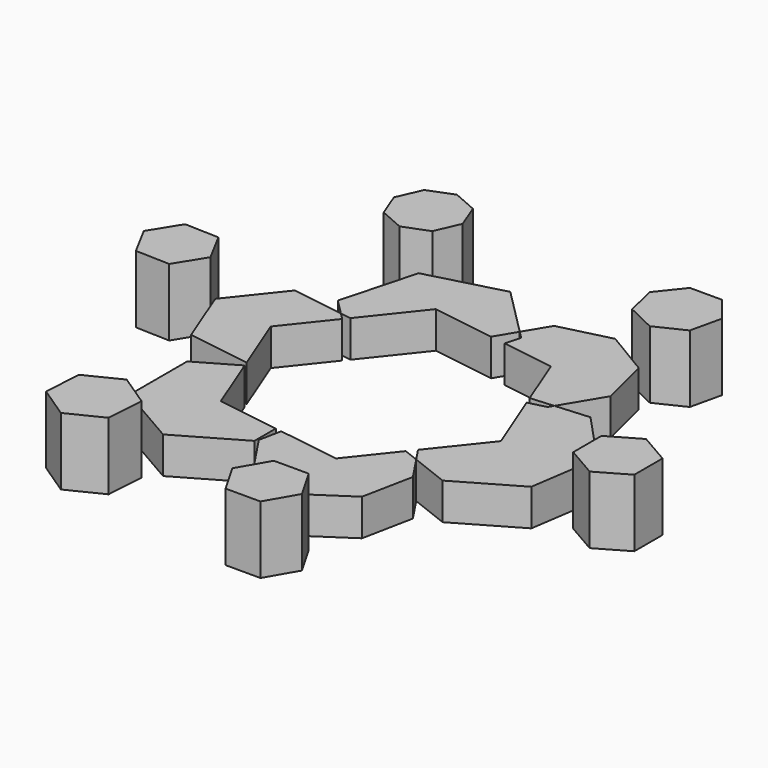
from build123d import *

# Parameters (mm, degrees)
F1_DEPTH = 25
F5_DEPTH = 46


# Not quite as in the source:
# - the program builds the solid bodies; features that only make, move or delete a surface that nothing else refers to are left out


with BuildPart() as f1:
    # F0 (on Top) → F1 (new body)
    with BuildSketch(Plane.XY):
        Polygon((222.1852089025, -548.7398207486), (222.1852089025, -530.5067178582), (179.5499098826, -524.1243193825), (163.7595795897, -484.0098680956), (136.9146108627, -499.5088180164), (136.9146108627, -548.7398207486), (179.5499098826, -573.3553221147), align=None)
    extrude(amount=F1_DEPTH)


with BuildPart() as f1b:
    # F0 (on Top) → F1, piece 2 (new body)
    with BuildSketch(Plane.XY):
        Polygon((119.4099858602, -474.2598081213), (162.4582974419, -480.7040335526), (146.5150045824, -440.2009894172), (170.8221101954, -409.6578891972), (166.217670693, -405.0340568941), (130.5717117228, -399.6979452818), (103.4666930007, -433.7567639858), align=None)
    extrude(amount=F1_DEPTH)


with BuildPart() as f1c:
    # F0 (on Top) → F1, piece 3 (new body)
    with BuildSketch(Plane.XY):
        Polygon((166.217670693, -405.0340568941), (173.6200233045, -406.1421707132), (202.6772876524, -369.6302572329), (245.5548420979, -376.0489207447), (253.9323629055, -362.0813747017), (221.2432641031, -329.2545972135), (169.6503089808, -342.9627487539), (155.7254388925, -394.4976343163), align=None)
    extrude(amount=F1_DEPTH)


with BuildPart() as f1d:
    # F0 (on Top) → F1, piece 4 (new body)
    with BuildSketch(Plane.XY):
        Polygon((258.9113491372, -367.0813312356), (256.0632308556, -377.6220004681), (291.8744760227, -382.982855014), (305.8703483184, -418.5385860855), (321.7506056308, -417.3324661794), (338.2210194956, -389.8719239393), (329.5177385501, -355.0822071929), (298.763544948, -336.6363115411), (263.9738282016, -345.3395924866), (253.9323629055, -362.0813747017), align=None)
    extrude(amount=F1_DEPTH)


with BuildPart() as f1e:
    # F0 (on Top) → F1, piece 5 (new body)
    with BuildSketch(Plane.XY):
        Polygon((324.9093813229, -466.9061849793), (296.7051560656, -502.3462119564), (302.8987264088, -511.6312355413), (329.0845431676, -521.8780365199), (370.4912763382, -497.9163008296), (377.5739128611, -450.6033154129), (344.999082975, -415.5667232977), (321.7506056308, -417.3324661794), (319.7751238438, -420.6261175414), (307.8649156693, -423.605672926), align=None)
    extrude(amount=F1_DEPTH)


with BuildPart() as f1f:
    # F0 (on Top) → F1, piece 6 (new body)
    with BuildSketch(Plane.XY):
        Polygon((268.7470982529, -537.4769171636), (226.4152229627, -531.1399404674), (223.3535547567, -546.4694037319), (243.0076640568, -575.933647824), (277.7395848212, -582.8704606597), (307.2038289133, -563.2163513596), (314.140641749, -528.4844305953), (302.8987264088, -511.6312355413), (292.541328463, -507.5782706716), align=None)
    extrude(amount=F1_DEPTH)


with BuildPart() as f5:
    # F4 (on Top) → F5 (new body)
    with BuildSketch(Plane.XY):
        Polygon((50.0373041585, -427.8748940379), (61.0507631347, -448.4392095655), (84.3667122812, -449.1834320724), (96.6692024515, -429.3633390516), (85.6557434752, -408.7990235239), (62.3397943287, -408.0548010171), align=None)
    extrude(amount=F5_DEPTH)


with BuildPart() as f5b:
    # F4 (on Top) → F5, piece 2 (new body)
    with BuildSketch(Plane.XY):
        Polygon((137.167817033, -297.5910984255), (129.8400703304, -314.3133761923), (136.4830069519, -331.3193115823), (153.2052847187, -338.647058285), (170.2112201088, -332.0041216635), (177.5389668114, -315.2818438967), (170.8960301899, -298.2759085066), (154.1737524231, -290.948161804), align=None)
    extrude(amount=F5_DEPTH)


with BuildPart() as f5c:
    # F4 (on Top) → F5, piece 3 (new body)
    with BuildSketch(Plane.XY):
        Polygon((429.8605322838, -484.2521358655), (429.8605322838, -460.1862620189), (409.0188741684, -448.1533250956), (388.177216053, -460.1862620189), (388.177216053, -484.2521358655), (409.0188741684, -496.2850727887), align=None)
    extrude(amount=F5_DEPTH)


with BuildPart() as f5d:
    # F4 (on Top) → F5, piece 4 (new body)
    with BuildSketch(Plane.XY):
        Polygon((269.8167730025, -632.8309774399), (293.5725879022, -632.8309774399), (305.450495352, -612.2578382492), (293.5725879022, -591.6846990585), (269.8167730025, -591.6846990585), (257.9388655527, -612.2578382492), align=None)
    extrude(amount=F5_DEPTH)


with BuildPart() as f5e:
    # F4 (on Top) → F5, piece 5 (new body)
    with BuildSketch(Plane.XY):
        Polygon((125.04553228, -605.0311075118), (146.7024442616, -619.4845689866), (170.0479650622, -607.9558637804), (171.7365738812, -581.9736970994), (150.0796618995, -567.5202356246), (126.7341410989, -579.0489408308), align=None)
    extrude(amount=F5_DEPTH)


with BuildPart() as f5f:
    # F4 (on Top) → F5, piece 6 (new body)
    with BuildSketch(Plane.XY):
        Polygon((340.1645370866, -297.4101305008), (318.3130076979, -297.4101305008), (304.688801969, -314.494344117), (309.551224697, -335.7980100419), (329.2387723923, -345.2790333185), (348.9263200876, -335.7980100419), (353.7887428155, -314.494344117), align=None)
    extrude(amount=F5_DEPTH)


solid = Compound([f1.part, f1b.part, f1c.part, f1d.part, f1e.part, f1f.part, f5.part, f5b.part, f5c.part, f5d.part, f5e.part, f5f.part])
